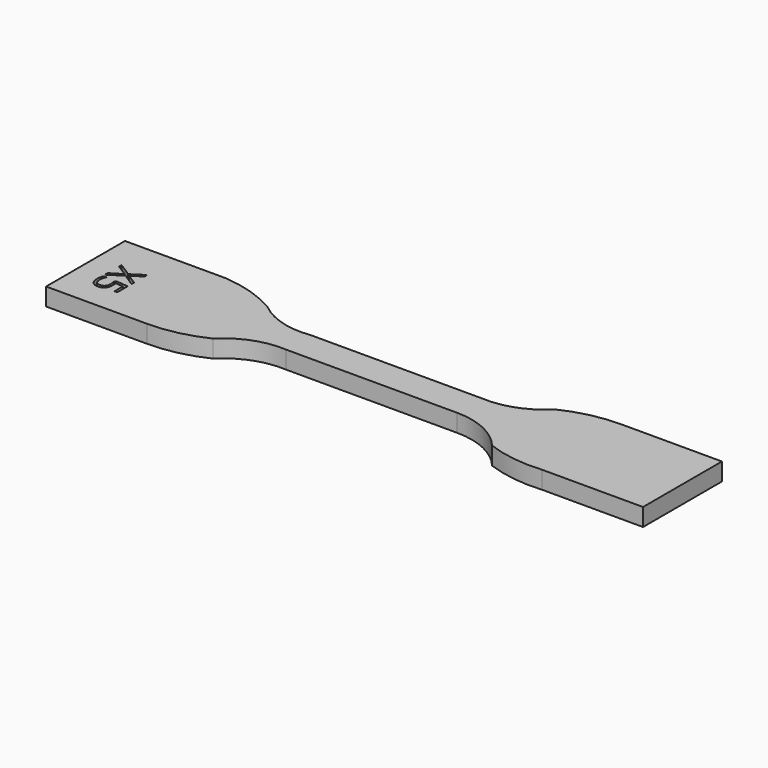
from build123d import *

# Parameters (mm, degrees)
F1_DEPTH     = 3.4
F2_TEXT_SIZE = 7.0564552314
F3_DEPTH     = 1


# Not quite as in the source:
# - Text() gives the source's letters only with a copy of the font that has no kerning and outlines rounded to 1/6400 em; it was checked with that copy


with BuildPart() as f1:
    # F0 (on Top) → F1 (new body)
    with BuildSketch(Plane.XY):
        with BuildLine():
            Line((-14.4320548165, 19.7811394548), (-33.8720548165, 19.7811394548))
            Line((-33.8720548165, 19.7811394548), (-33.8720548165, 0.7811394548))
            Line((-33.8720548165, 0.7811394548), (-14.4320548165, 0.7811394548))
            ThreePointArc((-14.4320548165, 0.7811394548), (-8.9053122052, 1.3996892086), (-3.6520548165, 3.2247301661))
            ThreePointArc((-3.6520548165, 3.2247301661), (1.3014698263, 6.4128780055), (7.1279451835, 7.2811394548))
            Line((7.1279451835, 7.2811394548), (40.1279451835, 7.2811394548))
            ThreePointArc((40.1279451835, 7.2811394548), (46.0837574042, 5.9511158081), (50.9079451835, 2.2137538538))
            ThreePointArc((50.9079451835, 2.2137538538), (56.2191047011, 0.9041953221), (61.6879451835, 0.7811394548))
            Line((61.6879451835, 0.7811394548), (81.1279451835, 0.7811394548))
            Line((81.1279451835, 0.7811394548), (81.1279451835, 19.7811394548))
            Line((81.1279451835, 19.7811394548), (61.6879451835, 19.7811394548))
            ThreePointArc((61.6879451835, 19.7811394548), (56.1612025723, 19.162589701), (50.9079451835, 17.3375487435))
            ThreePointArc((50.9079451835, 17.3375487435), (45.9544205407, 14.1494009041), (40.1279451835, 13.2811394548))
            Line((40.1279451835, 13.2811394548), (7.1279451835, 13.2811394548))
            ThreePointArc((7.1279451835, 13.2811394548), (1.4167452884, 13.6925537245), (-3.6520548165, 16.3560723447))
            ThreePointArc((-3.6520548165, 16.3560723447), (-8.8458057958, 18.686276846), (-14.4320548165, 19.7811394548))
        make_face()
    extrude(amount=F1_DEPTH)

    # F2 (on face) → F3 (cut)
    with BuildSketch(Plane.XY.offset(3.4)):
        with Locations(Location((-29.3720550835, 13.353464842), (0, 0, -90))):
            Text('X5', F2_TEXT_SIZE, font='Open Sans', text_align=(TextAlign.LEFT, TextAlign.BOTTOM))
    extrude(amount=-F3_DEPTH, mode=Mode.SUBTRACT)


solid = f1.part
